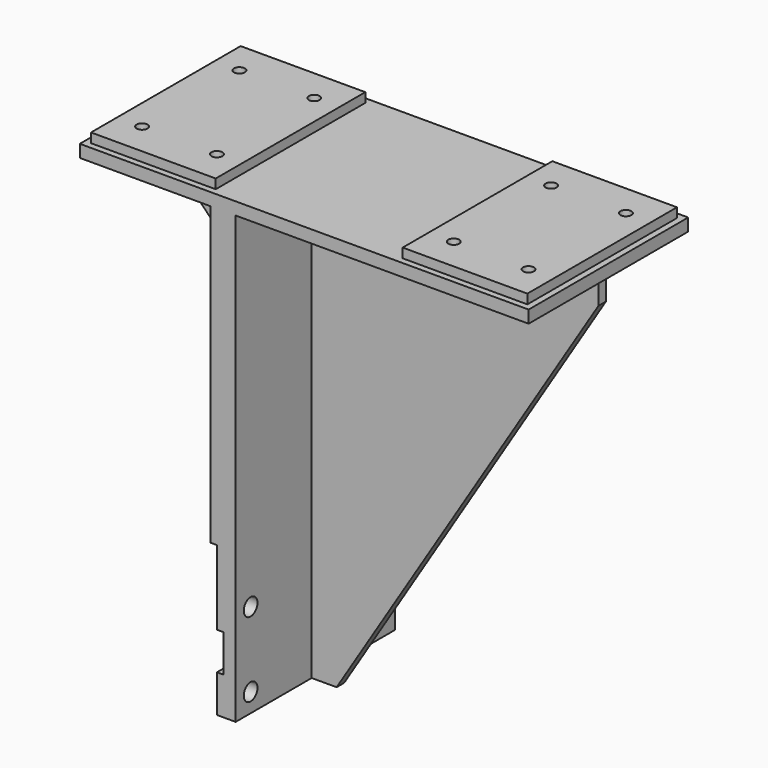
from build123d import *

# Parameters (mm, degrees)
F0_W      = 203.2
F0_H      = 454.152
F1_DEPTH  = 25.4
F2_W      = 6.35
F2_H      = 152.4
F3_DEPTH  = 203.201
F4_W      = 457.2
F4_H      = 203.2
F5_DEPTH  = 12.7
F6_W      = 127
F6_H      = 190.5
F7_DEPTH  = 9.652
F9_D      = 11.1125
F11_DEPTH = 4.7625
F12_W     = 38.1
F12_H     = 38.1
F13_DEPTH = 203.201
F15_D     = 17.4625
F17_DEPTH = 4.826


# Not quite as in the source:
# - a length typed as a fraction of an inch, garbled in the dataset ("3 / 203.2 mm" for 3/8 in), is restored


with BuildPart() as f1:
    # F0 (on Right) → F1 (new body)
    with BuildSketch(Plane.YZ):
        Rectangle(F0_W, F0_H)
    extrude(amount=F1_DEPTH)

    # F2 (on face) → F3 (cut, through all)
    with BuildSketch(Plane.XZ.offset(101.6)):
        with Locations((3.175, -150.876)):
            Rectangle(F2_W, F2_H)
    extrude(amount=-F3_DEPTH, mode=Mode.SUBTRACT)

    # F4 (on face) → F5 (join)
    with BuildSketch(Plane.XY.offset(227.076)):
        with Locations((95.25, 0)):
            Rectangle(F4_W, F4_H)
    extrude(amount=F5_DEPTH)

    # F6 (on face) → F7 (join)
    with BuildSketch(Plane.XY.offset(239.776)):
        with Locations((-63.5, 0)):
            Rectangle(F6_W, F6_H)
        with Locations((254, 0)):
            Rectangle(F6_W, F6_H)
    extrude(amount=F7_DEPTH)

    # F9 (through all)
    with Locations(Plane.XY.offset(249.428)):
        with Locations((-101.6, 61.976), (-25.4, 61.976), (-101.6, -61.976), (-25.4, -61.976), (215.9, 61.976), (292.1, 61.976), (215.9, -61.976), (292.1, -61.976)):
            Hole(F9_D / 2)

    # F10 (on Front) → F11 (join, symmetric)
    with BuildSketch(Plane.XZ):
        Polygon((317.5, 227.076), (25.4, 227.076), (25.4, -227.076), (50.8, -227.076), (317.5, 201.676), align=None)
    extrude(amount=F11_DEPTH, both=True)

    # F12 (on face) → F13 (cut, through all)
    with BuildSketch(Plane.XZ.offset(101.6)):
        with Locations((-5.842, -169.672)):
            Rectangle(F12_W, F12_H)
    extrude(amount=-F13_DEPTH, mode=Mode.SUBTRACT)

    # F15 (through all)
    with Locations(Plane(origin=(6.35, 0, 0), x_dir=(0, -1, 0), z_dir=(-1, 0, 0))):
        with Locations((-82.55, -131.572), (82.55, -131.572), (82.55, -207.772), (-82.55, -207.772)):
            Hole(F15_D / 2)

    # F16 (on Front) → F17 (join, symmetric)
    with BuildSketch(Plane.XZ):
        Polygon((0, 100.076), (0, 227.076), (-127, 227.076), (-127, 201.676), (-25.4, 100.076), align=None)
    extrude(amount=F17_DEPTH, both=True)


solid = f1.part
